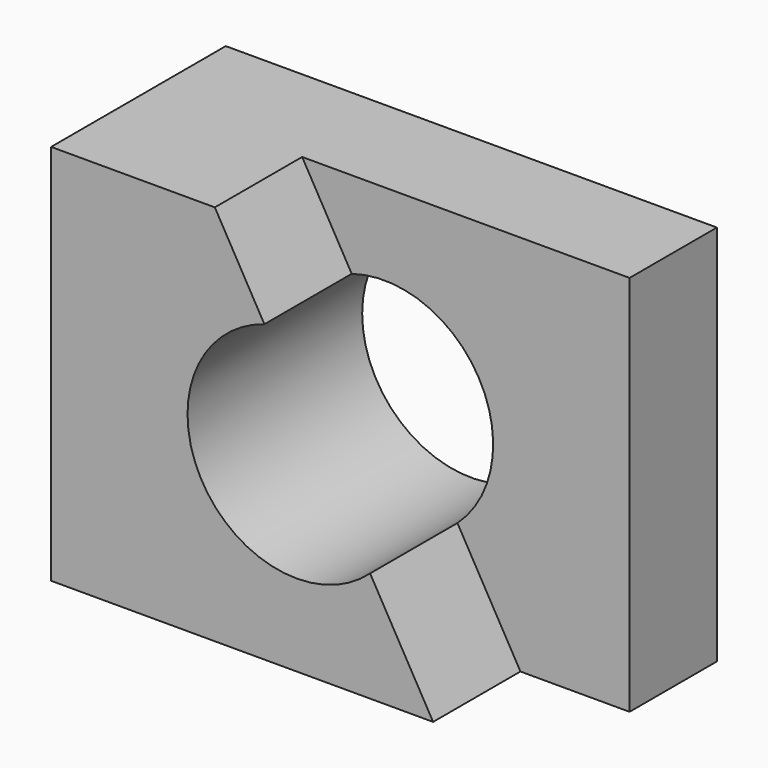
from build123d import *

# Parameters (mm, degrees)
F0_W     = 114.3
F0_H     = 88.9
F1_DEPTH = 25.4
F3_DEPTH = 25.4
F4_R     = 25.4
F5_DEPTH = 50.801


# Not quite as in the source:
# - a feature names something its author has since deleted; it is built from what else it names


with BuildPart() as f1:
    # F0 (on Front) → F1 (new body)
    with BuildSketch(Plane.XZ):
        with Locations((0, -6.6255477227)):
            Rectangle(F0_W, F0_H)
    extrude(amount=F1_DEPTH)

    # F2 (on face) → F3 (join)
    with BuildSketch(Plane.XZ.offset(25.4)):
        Polygon((31.75, -51.0755477227), (-19.05, 37.8244522773), (-57.15, 37.8244522773), (-57.15, -51.0755477227), align=None)
    extrude(amount=F3_DEPTH)

    # F4 (on face) → F5 (cut, through all)
    with BuildSketch(Plane(origin=(0, 0, 0), x_dir=(-1, 0, 0), z_dir=(0, 1, 0))):
        with Locations((0, -6.6255477227)):
            Circle(F4_R)
    extrude(amount=-F5_DEPTH, mode=Mode.SUBTRACT)


solid = f1.part
